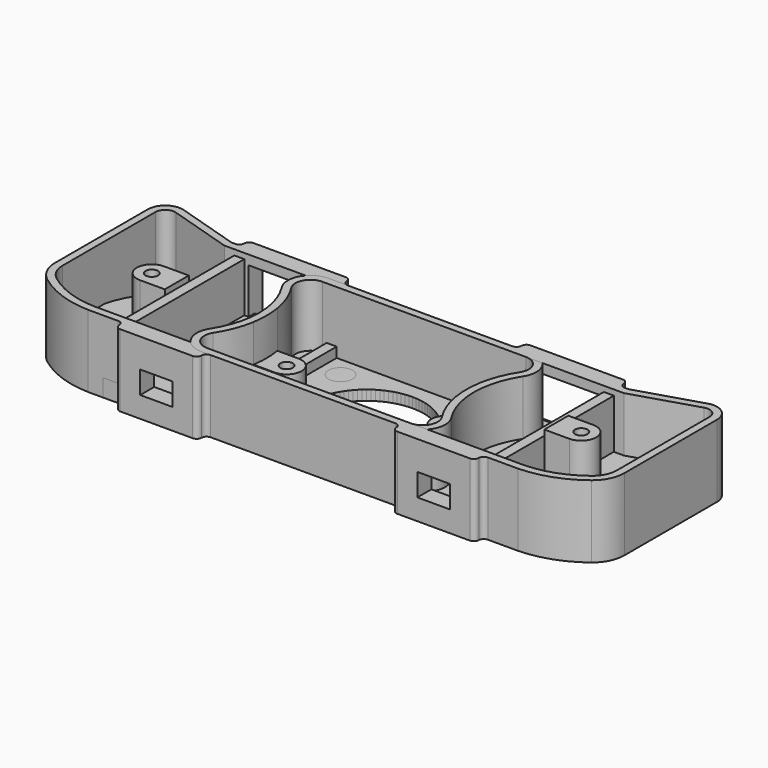
from build123d import *

# Parameters (mm, degrees)
F0_W      = 14.5
F0_H      = 2
F0_W_2    = 3
F0_W_3    = 5
F0_W_4    = 6.5
F0_R      = 11.5
F0_R_2    = 2.4
F0_H_2    = 1.5
F0_R_3    = 1.25
F0_W_5    = 2
F0_H_3    = 28.8
F1_DEPTH  = 2
F2_DEPTH  = 1.5
F3_DEPTH  = 11.4
F4_DEPTH  = 2
F5_DEPTH  = 12.5
F6_DEPTH  = 1
F7_W      = 6.5
F7_H      = 4.5
F8_DEPTH  = 25
F9_W      = 14.8
F9_H      = 10.2
F10_DEPTH = 25
F11_R     = 0.99999
F12_DEPTH = 5
F13_SIZE  = 0.5


# Not quite as in the source:
# - a fillet or chamfer is up to 0.001 mm smaller than in the source, because OpenCascade refuses the exact size


with BuildPart() as f1:
    # F0 (on Top) → F1 (new body)
    with BuildSketch(Plane.XY):
        with BuildLine():
            Line((-52.9083647375, 18.39742908), (-40, 14.4))
            Line((-40, 14.4), (-38, 14.4))
            Line((-38, 14.4), (-36, 14.4))
            Line((-36, 14.4), (-35, 14.4))
            Line((-35, 14.4), (-35, 15.9))
            Line((-35, 15.9), (-38, 15.9))
            Line((-38, 15.9), (-39.773058325, 15.9))
            Line((-39.773058325, 15.9), (-52.4646382907, 19.8302957313))
            ThreePointArc((-52.4646382907, 19.8302957313), (-55.5768045187, 19.3041876256), (-57, 16.4869402116))
            Line((-57, 16.4869402116), (-57, 14.4))
            Line((-57, 14.4), (-57, -6.6854864647))
            ThreePointArc((-57, -6.6854864647), (-56.3355938179, -9.5483250547), (-54.4782016024, -11.8259059039))
            ThreePointArc((-54.4782016024, -11.8259059039), (-49.0741349685, -14.7789093982), (-43.0187801742, -15.9))
            Line((-43.0187801742, -15.9), (-36, -15.9))
            Line((-36, -15.9), (-31, -15.9))
            Line((-31, -15.9), (-31, -14.4))
            Line((-31, -14.4), (-36, -14.4))
            Line((-36, -14.4), (-38, -14.4))
            Line((-38, -14.4), (-43, -14.4))
            ThreePointArc((-43, -14.4), (-48.5801604525, -13.3625487975), (-53.5601550788, -10.6396552641))
            ThreePointArc((-53.5601550788, -10.6396552641), (-54.9889183215, -8.8876699954), (-55.5, -6.6854864647))
            Line((-55.5, -6.6854864647), (-55.5, 14.4))
            Line((-55.5, 14.4), (-55.5, 16.4869402116))
            ThreePointArc((-55.5, 16.4869402116), (-54.6867454392, 18.0967958767), (-52.9083647375, 18.39742908))
        make_face()
        with BuildLine():
            Line((-20.5, 15.9), (-20.5, 14.4))
            Line((-20.5, 14.4), (-19.5, 14.4))
            Line((-19.5, 14.4), (-17.5, 14.4))
            Line((-17.5, 14.4), (20, 14.4))
            Line((20, 14.4), (20.363673852, 14.4))
            ThreePointArc((20.363673852, 14.4), (22.9986040489, 12.8342743312), (22.883149016, 9.7714285714))
            ThreePointArc((22.883149016, 9.7714285714), (21.2222885387, 6.5198464799), (20.2517606507, 3))
            ThreePointArc((20.2517606507, 3), (20, 0), (20.2517606507, -3))
            ThreePointArc((20.2517606507, -3), (21.2222885387, -6.5198464799), (22.883149016, -9.7714285714))
            ThreePointArc((22.883149016, -9.7714285714), (22.9986040489, -12.8342743312), (20.363673852, -14.4))
            Line((20.363673852, -14.4), (20, -14.4))
            Line((20, -14.4), (-17.5, -14.4))
            Line((-17.5, -14.4), (-19.5, -14.4))
            Line((-19.5, -14.4), (-24.5, -14.4))
            Line((-24.5, -14.4), (-24.5, -15.9))
            Line((-24.5, -15.9), (-19.5, -15.9))
            Line((-19.5, -15.9), (20, -15.9))
            Line((20, -15.9), (20.363673852, -15.9))
            ThreePointArc((20.363673852, -15.9), (24.3160691474, -13.5514114968), (24.142886598, -8.9571428571))
            ThreePointArc((24.142886598, -8.9571428571), (21.5, 0), (24.142886598, 8.9571428571))
            ThreePointArc((24.142886598, 8.9571428571), (24.3160691474, 13.5514114968), (20.363673852, 15.9))
            Line((20.363673852, 15.9), (20, 15.9))
            Line((20, 15.9), (-17.5, 15.9))
            Line((-17.5, 15.9), (-20.5, 15.9))
        make_face()
        with Locations((-27.75, 16.9)):
            Rectangle(F0_W, F0_H)
        with Locations((-36.5, 16.9)):
            Rectangle(F0_W_2, F0_H)
        with Locations((-19, 16.9)):
            Rectangle(F0_W_2, F0_H)
        with Locations((-33.5, -16.9)):
            Rectangle(F0_W_3, F0_H)
        with Locations((-27.75, -16.9)):
            Rectangle(F0_W_4, F0_H)
        with Locations((-22, -16.9)):
            Rectangle(F0_W_3, F0_H)
        with BuildLine():
            Line((40.1, 15.9), (20.363673852, 15.9))
            ThreePointArc((20.363673852, 15.9), (24.3160691474, 13.5514114968), (24.142886598, 8.9571428571))
            ThreePointArc((24.142886598, 8.9571428571), (21.5, 0), (24.142886598, -8.9571428571))
            ThreePointArc((24.142886598, -8.9571428571), (24.3160691474, -13.5514114968), (20.363673852, -15.9))
            Line((20.363673852, -15.9), (40.1, -15.9))
            ThreePointArc((40.1, -15.9), (24.2, 0), (40.1, 15.9))
        make_face()
        with BuildLine():
            ThreePointArc((56, 0), (51.3429978209, 11.2429978209), (40.1, 15.9))
            ThreePointArc((40.1, 15.9), (24.2, 0), (40.1, -15.9))
            ThreePointArc((40.1, -15.9), (51.3429978209, -11.2429978209), (56, 0))
        make_face()
        with BuildLine():
            Line((20, 14.4), (-17.5, 14.4))
            Line((-17.5, 14.4), (-17.5, -14.4))
            Line((-17.5, -14.4), (20, -14.4))
            Line((20, -14.4), (20.363673852, -14.4))
            ThreePointArc((20.363673852, -14.4), (22.9986040489, -12.8342743312), (22.883149016, -9.7714285714))
            ThreePointArc((22.883149016, -9.7714285714), (21.2222885387, -6.5198464799), (20.2517606507, -3))
            Line((20.2517606507, -3), (16, -3))
            ThreePointArc((16, -3), (13, 0), (16, 3))
            Line((16, 3), (20.2517606507, 3))
            ThreePointArc((20.2517606507, 3), (21.2222885387, 6.5198464799), (22.883149016, 9.7714285714))
            ThreePointArc((22.883149016, 9.7714285714), (22.9986040489, 12.8342743312), (20.363673852, 14.4))
            Line((20.363673852, 14.4), (20, 14.4))
        make_face()
        Circle(F0_R, mode=Mode.SUBTRACT)
        with Locations((13.486796875, 10.3492178474)):
            Circle(F0_R_2, mode=Mode.SUBTRACT)
        with Locations((-27.75, 15.15)):
            Rectangle(F0_W, F0_H_2)
        Polygon((-35, 14.4), (-36, 14.4), (-36, -14.4), (-31, -14.4), (-24.5, -14.4), (-19.5, -14.4), (-19.5, 14.4), (-20.5, 14.4), align=None)
        Polygon((-36, 14.4), (-38, 14.4), (-38, 3), (-38, -3), (-38, -14.4), (-36, -14.4), align=None)
        with BuildLine():
            Line((-38, -3), (-38, 3))
            Line((-38, 3), (-43, 3))
            ThreePointArc((-43, 3), (-46, 0), (-43, -3))
            Line((-43, -3), (-38, -3))
        make_face()
        with Locations((-43, 0)):
            Circle(F0_R_3, mode=Mode.SUBTRACT)
        with BuildLine():
            Line((-38, 14.4), (-40, 14.4))
            Line((-40, 14.4), (-52.9083647375, 18.39742908))
            ThreePointArc((-52.9083647375, 18.39742908), (-54.6867454392, 18.0967958767), (-55.5, 16.4869402116))
            Line((-55.5, 16.4869402116), (-55.5, 14.4))
            Line((-55.5, 14.4), (-55.5, -6.6854864647))
            ThreePointArc((-55.5, -6.6854864647), (-54.9889183215, -8.8876699954), (-53.5601550788, -10.6396552641))
            ThreePointArc((-53.5601550788, -10.6396552641), (-48.5801604525, -13.3625487975), (-43, -14.4))
            Line((-43, -14.4), (-38, -14.4))
            Line((-38, -14.4), (-38, -3))
            Line((-38, -3), (-43, -3))
            ThreePointArc((-43, -3), (-46, 0), (-43, 3))
            Line((-43, 3), (-38, 3))
            Line((-38, 3), (-38, 14.4))
        make_face()
        with Locations((-18.5, 0)):
            Rectangle(F0_W_5, F0_H_3)
        with BuildLine():
            ThreePointArc((20.2517606507, -3), (20, 0), (20.2517606507, 3))
            Line((20.2517606507, 3), (16, 3))
            ThreePointArc((16, 3), (13, 0), (16, -3))
            Line((16, -3), (20.2517606507, -3))
        make_face()
        with Locations((16, 0)):
            Circle(F0_R_3, mode=Mode.SUBTRACT)
        with Locations((-27.75, -15.15)):
            Rectangle(F0_W_4, F0_H_2)
    extrude(amount=-F1_DEPTH)

    # F0 (on Top) → F2 (join)
    with BuildSketch(Plane.XY):
        with BuildLine():
            Line((40.1, 15.9), (20.363673852, 15.9))
            ThreePointArc((20.363673852, 15.9), (24.3160691474, 13.5514114968), (24.142886598, 8.9571428571))
            ThreePointArc((24.142886598, 8.9571428571), (21.5, 0), (24.142886598, -8.9571428571))
            ThreePointArc((24.142886598, -8.9571428571), (24.3160691474, -13.5514114968), (20.363673852, -15.9))
            Line((20.363673852, -15.9), (40.1, -15.9))
            ThreePointArc((40.1, -15.9), (24.2, 0), (40.1, 15.9))
        make_face()
        with BuildLine():
            ThreePointArc((56, 0), (51.3429978209, 11.2429978209), (40.1, 15.9))
            ThreePointArc((40.1, 15.9), (24.2, 0), (40.1, -15.9))
            ThreePointArc((40.1, -15.9), (51.3429978209, -11.2429978209), (56, 0))
        make_face()
    extrude(amount=F2_DEPTH)

    # F0 (on Top) → F3 (join)
    with BuildSketch(Plane.XY):
        Polygon((-36, 14.4), (-38, 14.4), (-38, 3), (-38, -3), (-38, -14.4), (-36, -14.4), align=None)
    extrude(amount=F3_DEPTH)

    # F0 (on Top) → F4 (join)
    with BuildSketch(Plane.XY):
        with Locations((-18.5, 0)):
            Rectangle(F0_W_5, F0_H_3)
    extrude(amount=F4_DEPTH)

    # F0 (on Top) → F5 (join)
    with BuildSketch(Plane.XY):
        with BuildLine():
            Line((-20.5, 15.9), (-20.5, 14.4))
            Line((-20.5, 14.4), (-19.5, 14.4))
            Line((-19.5, 14.4), (-17.5, 14.4))
            Line((-17.5, 14.4), (20, 14.4))
            Line((20, 14.4), (20.363673852, 14.4))
            ThreePointArc((20.363673852, 14.4), (22.9986040489, 12.8342743312), (22.883149016, 9.7714285714))
            ThreePointArc((22.883149016, 9.7714285714), (21.2222885387, 6.5198464799), (20.2517606507, 3))
            ThreePointArc((20.2517606507, 3), (20, 0), (20.2517606507, -3))
            ThreePointArc((20.2517606507, -3), (21.2222885387, -6.5198464799), (22.883149016, -9.7714285714))
            ThreePointArc((22.883149016, -9.7714285714), (22.9986040489, -12.8342743312), (20.363673852, -14.4))
            Line((20.363673852, -14.4), (20, -14.4))
            Line((20, -14.4), (-17.5, -14.4))
            Line((-17.5, -14.4), (-19.5, -14.4))
            Line((-19.5, -14.4), (-24.5, -14.4))
            Line((-24.5, -14.4), (-24.5, -15.9))
            Line((-24.5, -15.9), (-19.5, -15.9))
            Line((-19.5, -15.9), (20, -15.9))
            Line((20, -15.9), (20.363673852, -15.9))
            ThreePointArc((20.363673852, -15.9), (24.3160691474, -13.5514114968), (24.142886598, -8.9571428571))
            ThreePointArc((24.142886598, -8.9571428571), (21.5, 0), (24.142886598, 8.9571428571))
            ThreePointArc((24.142886598, 8.9571428571), (24.3160691474, 13.5514114968), (20.363673852, 15.9))
            Line((20.363673852, 15.9), (20, 15.9))
            Line((20, 15.9), (-17.5, 15.9))
            Line((-17.5, 15.9), (-20.5, 15.9))
        make_face()
        with BuildLine():
            Line((-52.9083647375, 18.39742908), (-40, 14.4))
            Line((-40, 14.4), (-38, 14.4))
            Line((-38, 14.4), (-36, 14.4))
            Line((-36, 14.4), (-35, 14.4))
            Line((-35, 14.4), (-35, 15.9))
            Line((-35, 15.9), (-38, 15.9))
            Line((-38, 15.9), (-39.773058325, 15.9))
            Line((-39.773058325, 15.9), (-52.4646382907, 19.8302957313))
            ThreePointArc((-52.4646382907, 19.8302957313), (-55.5768045187, 19.3041876256), (-57, 16.4869402116))
            Line((-57, 16.4869402116), (-57, 14.4))
            Line((-57, 14.4), (-57, -6.6854864647))
            ThreePointArc((-57, -6.6854864647), (-56.3355938179, -9.5483250547), (-54.4782016024, -11.8259059039))
            ThreePointArc((-54.4782016024, -11.8259059039), (-49.0741349685, -14.7789093982), (-43.0187801742, -15.9))
            Line((-43.0187801742, -15.9), (-36, -15.9))
            Line((-36, -15.9), (-31, -15.9))
            Line((-31, -15.9), (-31, -14.4))
            Line((-31, -14.4), (-36, -14.4))
            Line((-36, -14.4), (-38, -14.4))
            Line((-38, -14.4), (-43, -14.4))
            ThreePointArc((-43, -14.4), (-48.5801604525, -13.3625487975), (-53.5601550788, -10.6396552641))
            ThreePointArc((-53.5601550788, -10.6396552641), (-54.9889183215, -8.8876699954), (-55.5, -6.6854864647))
            Line((-55.5, -6.6854864647), (-55.5, 14.4))
            Line((-55.5, 14.4), (-55.5, 16.4869402116))
            ThreePointArc((-55.5, 16.4869402116), (-54.6867454392, 18.0967958767), (-52.9083647375, 18.39742908))
        make_face()
        with Locations((-33.5, -16.9)):
            Rectangle(F0_W_3, F0_H)
        with Locations((-22, -16.9)):
            Rectangle(F0_W_3, F0_H)
        with Locations((-27.75, -16.9)):
            Rectangle(F0_W_4, F0_H)
        with Locations((-27.75, -15.15)):
            Rectangle(F0_W_4, F0_H_2)
        with Locations((-36.5, 16.9)):
            Rectangle(F0_W_2, F0_H)
        with Locations((-27.75, 15.15)):
            Rectangle(F0_W, F0_H_2)
        with Locations((-27.75, 16.9)):
            Rectangle(F0_W, F0_H)
        with Locations((-19, 16.9)):
            Rectangle(F0_W_2, F0_H)
        with BuildLine():
            Line((-38, -3), (-38, 3))
            Line((-38, 3), (-43, 3))
            ThreePointArc((-43, 3), (-46, 0), (-43, -3))
            Line((-43, -3), (-38, -3))
        make_face()
        with Locations((-43, 0)):
            Circle(F0_R_3, mode=Mode.SUBTRACT)
    extrude(amount=F5_DEPTH)

    # F0 (on Top) → F6 (cut)
    with BuildSketch(Plane.XY):
        Polygon((-35, 14.4), (-36, 14.4), (-36, -14.4), (-31, -14.4), (-24.5, -14.4), (-19.5, -14.4), (-19.5, 14.4), (-20.5, 14.4), align=None)
    extrude(amount=-F6_DEPTH, mode=Mode.SUBTRACT)

    # F7 (on face) → F8 (cut)
    with BuildSketch(Plane.XZ.offset(17.9)):
        with Locations((-27.75, 4.45)):
            Rectangle(F7_W, F7_H)
    extrude(amount=-F8_DEPTH, mode=Mode.SUBTRACT)

    # F9 (on face) → F10 (cut)
    with BuildSketch(Plane(origin=(0, 17.9, 0), x_dir=(-1, 0, 0), z_dir=(0, 1, 0))):
        with Locations((27.75, 5.5)):
            Rectangle(F9_W, F9_H)
    extrude(amount=-F10_DEPTH, mode=Mode.SUBTRACT)

    # F11 (radius 1 in the source; OpenCascade refuses exactly that, so slightly less here)
    f11_edges = [f1.edges().sort_by_distance(p)[0] for p in [
        (-17.5, 17.9, 5.25),
        (-38, 17.9, 5.25),
        (-17.5, 15.9, 5.25),
        (-38, 15.9, 5.25),
        (-19.5, -17.9, 5.25),
        (-19.5, -15.9, 5.25),
        (-36, -15.9, 5.25),
        (-36, -17.9, 5.25),
    ]]
    fillet(f11_edges, radius=F11_R)

    # F0 (on Top) → F12 (join)
    with BuildSketch(Plane.XY):
        with BuildLine():
            ThreePointArc((20.2517606507, -3), (20, 0), (20.2517606507, 3))
            Line((20.2517606507, 3), (16, 3))
            ThreePointArc((16, 3), (13, 0), (16, -3))
            Line((16, -3), (20.2517606507, -3))
        make_face()
        with Locations((16, 0)):
            Circle(F0_R_3, mode=Mode.SUBTRACT)
    extrude(amount=F12_DEPTH)

    # F13
    f13_edges = [f1.edges().sort_by_distance(p)[0] for p in [
        (-44.25, 0, -2),
        (14.75, 0, -2),
    ]]
    chamfer(f13_edges, length=F13_SIZE)


with BuildPart() as f14_1:
    # F14: instance of F1
    add(f1.part.mirror(Plane.YZ))


solid = Compound([f1.part, f14_1.part])
